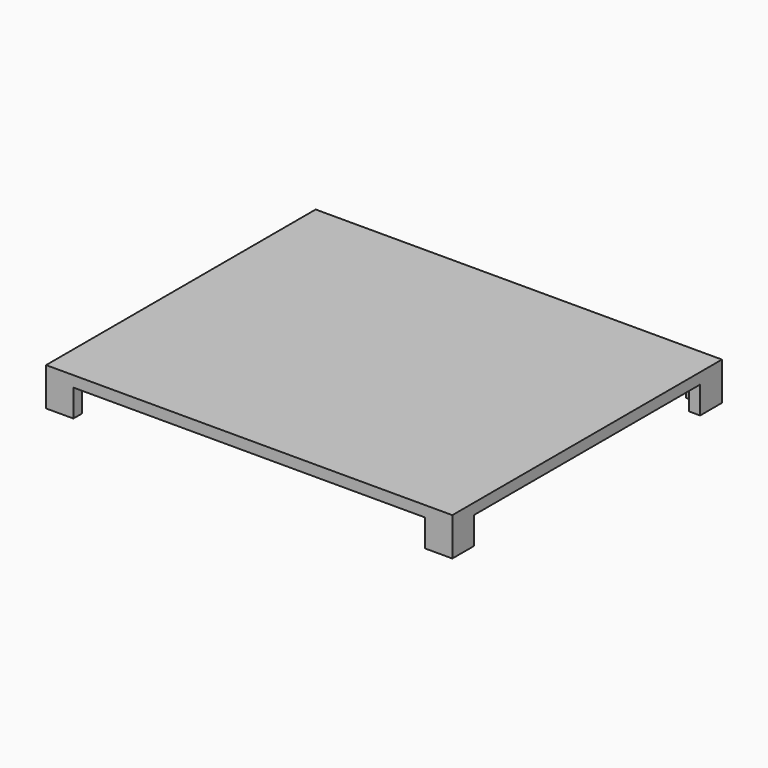
from build123d import *

# Parameters (mm, degrees)
F0_W     = 148.97
F0_H     = 123.57
F0_W_2   = 132.97
F0_H_2   = 107.57
F1_DEPTH = 4
F4_DEPTH = 10
F6_W     = 132.97
F6_H     = 107.57
F7_DEPTH = 4


# Not quite as in the source:
# - a pattern or mirror of a feature is missing from the dataset's text; its kind, count and spacing are read off the source's solid


with BuildPart() as f1:
    # F0 (on Top) → F1 (new body)
    with BuildSketch(Plane.XY):
        with Locations((70.485, -57.785)):
            Rectangle(F0_W, F0_H)
        with Locations((70.485, -57.785)):
            Rectangle(F0_W_2, F0_H_2, mode=Mode.SUBTRACT)
    extrude(amount=F1_DEPTH)

    # F2 (on face) → F4 (join)
    with BuildSketch(Plane(origin=(0, 0, 0), x_dir=(1, 0, 0), z_dir=(0, 0, -1))):
        Polygon((6, 119.57), (-4, 119.57), (-4, 109.57), (0, 109.57), (0, 115.57), (6, 115.57), align=None)
        Polygon((6, 0), (0, 0), (0, 6), (-4, 6), (-4, -4), (6, -4), align=None)
    f4 = extrude(amount=F4_DEPTH)

    # F4_copies: F4 across plane
    add(f4.mirror(Plane(origin=(70.485, 0, 0), x_dir=(0, 0, 1), z_dir=(1, 0, 0))))

    # F6 (on face) → F7 (join, through all)
    with BuildSketch(Plane.XY.offset(4)):
        with Locations((70.485, -57.785)):
            Rectangle(F6_W, F6_H)
    extrude(amount=-F7_DEPTH)


solid = f1.part
